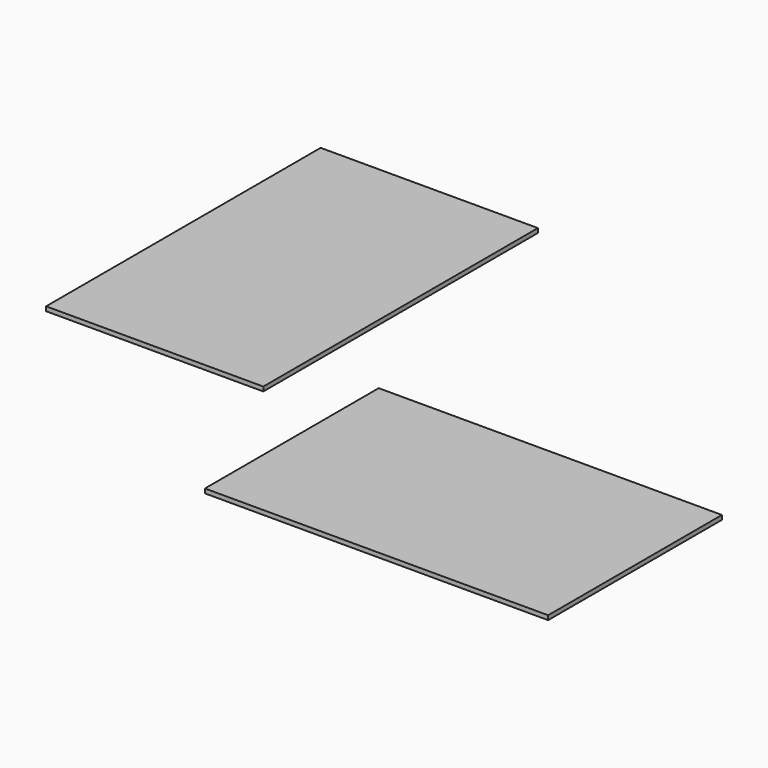
from build123d import *

# Parameters (mm, degrees)
F0_W     = 450
F0_H     = 25
F0_W_2   = 25
F0_H_2   = 740
F1_DEPTH = 10
F0_H_3   = 450
F0_W_3   = 740


# Not quite as in the source:
# - a feature names something its author has since deleted; it is built from what else it names


with BuildPart() as f1:
    # F0 (on Top) → F1 (new body)
    with BuildSketch(Plane.XY):
        Polygon((-1182.8998201413, 1223.8749871956), (-1182.8998201413, 953.8749871956), (-1182.8998201413, 653.8749871956), (-1182.8998201413, 483.8749871956), (-732.8998201413, 483.8749871956), (-732.8998201413, 1223.8749871956), align=None)
        Polygon((-1182.8998201413, 653.8749871956), (-1182.8998201413, 953.8749871956), (-1182.8998201413, 1223.8749871956), (-1182.8998201413, 1248.8749871956), (-1207.8998201413, 1248.8749871956), (-1207.8998201413, 483.8749871956), (-1182.8998201413, 483.8749871956), align=None)
        with Locations((-957.8998201413, 1236.3749871956)):
            Rectangle(F0_W, F0_H)
        with Locations((-957.8998201413, 471.3749871956)):
            Rectangle(F0_W, F0_H)
        with Locations((-1195.3998201413, 471.3749871956)):
            Rectangle(F0_W_2, F0_H)
        with Locations((-720.3998201413, 853.8749871956)):
            Rectangle(F0_W_2, F0_H_2)
        with Locations((-720.3998201413, 1236.3749871956)):
            Rectangle(F0_W_2, F0_H)
        with Locations((-720.3998201413, 471.3749871956)):
            Rectangle(F0_W_2, F0_H)
    extrude(amount=F1_DEPTH)


with BuildPart() as f1b:
    # F0 (on Top) → F1, piece 2 (new body)
    with BuildSketch(Plane.XY):
        Polygon((-517.0606966229, 108.5655740079), (-347.0606966229, 108.5655740079), (-47.0606966229, 108.5655740079), (222.9393033771, 108.5655740079), (222.9393033771, 558.5655740079), (-517.0606966229, 558.5655740079), align=None)
        Polygon((-47.0606966229, 108.5655740079), (-347.0606966229, 108.5655740079), (-517.0606966229, 108.5655740079), (-517.0606966229, 83.5655740079), (-309.5606966229, 83.5655740079), (-284.5606966229, 83.5655740079), (-9.5606966229, 83.5655740079), (15.4393033771, 83.5655740079), (247.9393033771, 83.5655740079), (247.9393033771, 108.5655740079), (222.9393033771, 108.5655740079), align=None)
        with Locations((-529.5606966229, 96.0655740079)):
            Rectangle(F0_W_2, F0_H)
        with Locations((-529.5606966229, 333.5655740079)):
            Rectangle(F0_W_2, F0_H_3)
        with Locations((235.4393033771, 333.5655740079)):
            Rectangle(F0_W_2, F0_H_3)
        with Locations((-147.0606966229, 571.0655740079)):
            Rectangle(F0_W_3, F0_H)
        with Locations((-529.5606966229, 571.0655740079)):
            Rectangle(F0_W_2, F0_H)
        with Locations((235.4393033771, 571.0655740079)):
            Rectangle(F0_W_2, F0_H)
    extrude(amount=F1_DEPTH)


solid = Compound([f1.part, f1b.part])
